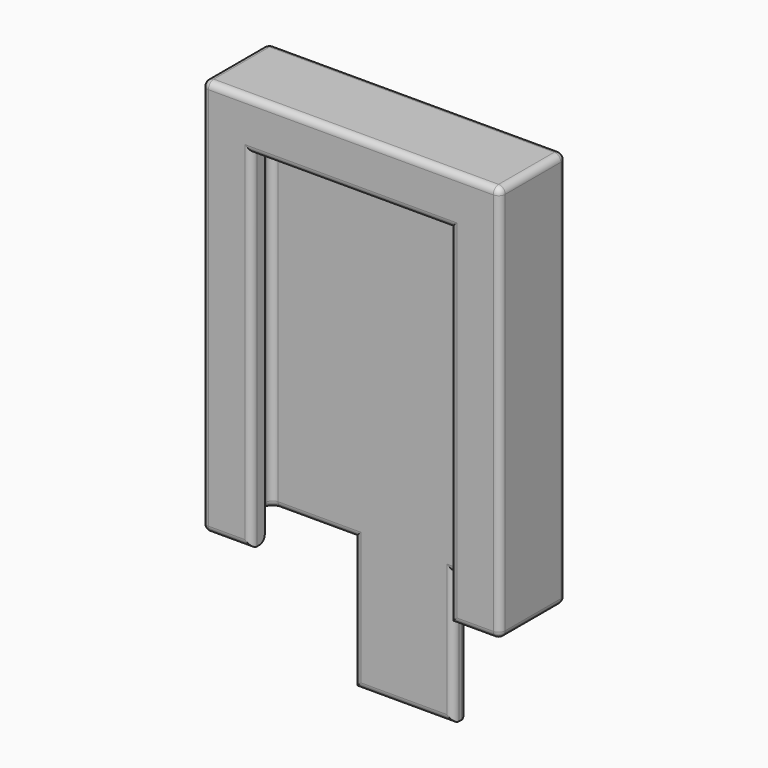
from build123d import *

# Parameters (mm, degrees)
F0_W     = 90
F0_H     = 25
F0_W_2   = 80
F0_H_2   = 15
F1_DEPTH = 120
F3_DEPTH = 110
F2_W     = 60
F2_H     = 105
F4_DEPTH = 10
F5_W     = 30
F5_H     = 40
F6_DEPTH = 5
F7_R     = 2


with BuildPart() as f1:
    # F0 (on Top) → F1 (new body)
    with BuildSketch(Plane.XY):
        Rectangle(F0_W, F0_H)
        Rectangle(F0_W_2, F0_H_2, mode=Mode.SUBTRACT)
        Rectangle(F0_W_2, F0_H_2)
    extrude(amount=F1_DEPTH)

    # F0 (on Top) → F3 (cut)
    with BuildSketch(Plane.XY):
        Rectangle(F0_W_2, F0_H_2)
    extrude(amount=F3_DEPTH, mode=Mode.SUBTRACT)

    # F2 (on face) → F4 (cut)
    with BuildSketch(Plane.XZ.offset(12.5)):
        with Locations((0, 52.5)):
            Rectangle(F2_W, F2_H)
    extrude(amount=-F4_DEPTH, mode=Mode.SUBTRACT)

    # F5 (on face) → F6 (join)
    with BuildSketch(Plane(origin=(0, 12.5, 0), x_dir=(-1, 0, 0), z_dir=(0, 1, 0))):
        with Locations((0, -20)):
            Rectangle(F5_W, F5_H)
    extrude(amount=-F6_DEPTH)

    # F7
    f7_edges = [f1.edges().sort_by_distance(p)[0] for p in [
        (40, 7.5, 55),
        (0, 7.5, 110),
        (-40, 7.5, 55),
        (-27.5, 7.5, 0),
        (-15, 7.5, -20),
        (0, 7.5, -40),
        (15, 7.5, -20),
        (27.5, 7.5, 0),
        (30, -7.5, 52.5),
        (-40, -7.5, 55),
        (-40, 0, 110),
        (0, -7.5, 110),
        (40, 0, 110),
        (-37.5, -12.5, 0),
        (-30, -12.5, 52.5),
        (0, -12.5, 105),
        (30, -12.5, 52.5),
        (37.5, -12.5, 0),
        (45, -12.5, 60),
        (0, -12.5, 120),
        (-45, -12.5, 60),
        (45, 12.5, 60),
        (45, 0, 0),
        (45, 0, 120),
        (0, 12.5, 120),
        (-45, 12.5, 60),
        (-30, 12.5, 0),
        (-15, 12.5, -20),
        (0, 12.5, -40),
        (15, 12.5, -20),
        (30, 12.5, 0),
        (-45, 0, 0),
        (-45, 0, 120),
        (-40, 0, 0),
        (-35, -7.5, 0),
        (40, 0, 0),
    ]]
    fillet(f7_edges, radius=F7_R)


solid = f1.part
